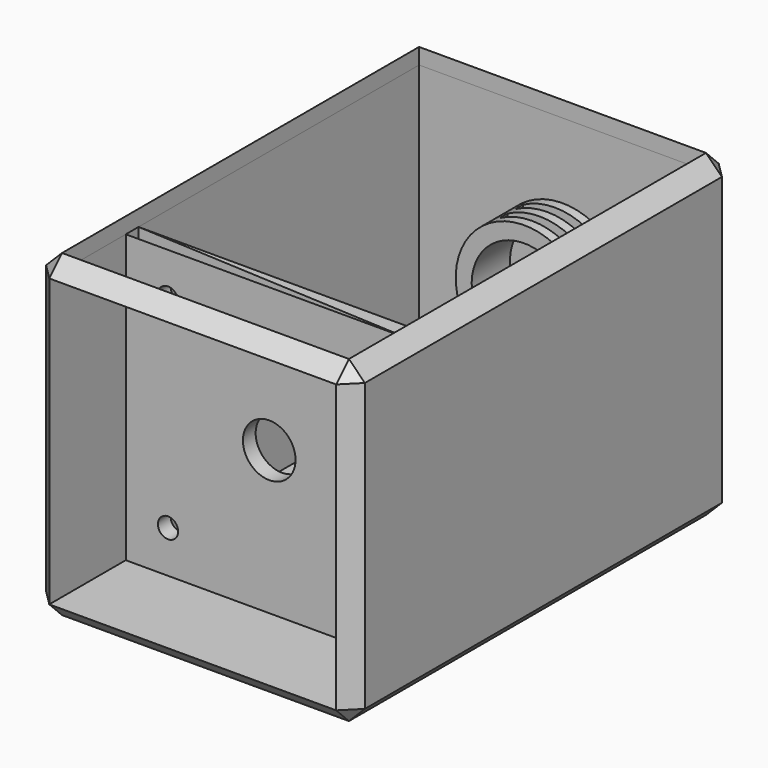
from build123d import *

# Parameters (mm, degrees)
F0_W           = 100
F0_H           = 100
F1_DEPTH       = 150
F2_W           = 90
F2_H           = 90
F3_DEPTH       = 145
F5_R           = 21.5
F5_R_2         = 16.5
F6_DEPTH       = 15
F8_DEPTH       = 21.7
F8_DEPTH_BACK  = 10
F10_W          = 3
F10_H          = 5
F11_DEPTH      = 5
F11_DEPTH_BACK = 4
F12_R          = 1
F13_DEPTH      = 15
F14_W          = 33
F14_H          = 43
F15_DEPTH      = 34
F17_DEPTH      = 130.001
F18_SIZE       = 4.99999
F19_W          = 90
F19_H          = 5
F20_DEPTH      = 90
F21_R          = 8.255
F22_DEPTH      = 5
F23_R          = 3.175
F24_DEPTH      = 5
F25_DEPTH      = 5


# Not quite as in the source:
# - a fillet or chamfer is up to 0.001 mm smaller than in the source, because OpenCascade refuses the exact size


with BuildPart() as f1:
    # F0 (on Front) → F1 (new body)
    with BuildSketch(Plane.XZ):
        Rectangle(F0_W, F0_H)
    extrude(amount=F1_DEPTH)

    # F2 (on face) → F3 (cut)
    with BuildSketch(Plane.XZ.offset(150)):
        Rectangle(F2_W, F2_H)
    extrude(amount=-F3_DEPTH, mode=Mode.SUBTRACT)

    # F5 (on face) → F6 (join)
    with BuildSketch(Plane.XZ.offset(5)):
        Circle(F5_R)
        Circle(F5_R_2, mode=Mode.SUBTRACT)
    extrude(amount=F6_DEPTH)

    # F7 (on Right) → F8 (cut, two sides)
    with BuildSketch(Plane.YZ) as f8_sk:
        Polygon((-8, 21.5), (-11, 21.5), (-11, 5), (-14, 5), (-14, 21.5), (-17, 21.5), (-17, -21.5), (-14, -21.5), (-14, 0), (-11, 0), (-11, -21.5), (-8, -21.5), align=None)
    extrude(amount=F8_DEPTH, mode=Mode.SUBTRACT)
    extrude(f8_sk.sketch, amount=-F8_DEPTH_BACK, mode=Mode.SUBTRACT)

    # F10 (on offset) → F11 (join, two sides)
    with BuildSketch(Plane.YZ.offset(21)) as f11_sk:
        with Locations((-12.5, 7.5)):
            Rectangle(F10_W, F10_H)
        with Locations((-12.5, -2.5)):
            Rectangle(F10_W, F10_H)
    extrude(amount=F11_DEPTH)
    extrude(f11_sk.sketch, amount=-F11_DEPTH_BACK)

    # F12 (on face) → F13 (cut, through all)
    with BuildSketch(Plane.XY.offset(10)):
        with Locations((23, -12.5)):
            Circle(F12_R)
    extrude(amount=-F13_DEPTH, mode=Mode.SUBTRACT)

    # F14 (on face) → F15 (join)
    with BuildSketch(Plane.XY.offset(-45)):
        with Locations((0, -41.5)):
            Rectangle(F14_W, F14_H)
    extrude(amount=F15_DEPTH)

    # F16 (on face) → F17 (cut, through all)
    with BuildSketch(Plane(origin=(0, -20, 0), x_dir=(-1, 0, 0), z_dir=(0, 1, 0))):
        with BuildLine():
            Line((12.2983738762, -11), (-12.2983738762, -11))
            ThreePointArc((-12.2983738762, -11), (0, -16.5), (12.2983738762, -11))
        make_face()
    extrude(amount=-F17_DEPTH, mode=Mode.SUBTRACT)

    # F18 (size 5 in the source; OpenCascade refuses exactly that, so slightly less here)
    f18_edges = [f1.edges().sort_by_distance(p)[0] for p in [
        (50, -75, 50),
        (-50, -75, 50),
        (0, 0, 50),
        (0, -150, 50),
        (50, -75, -50),
        (50, 0, 0),
        (50, -150, 0),
        (-50, -75, -50),
        (0, 0, -50),
        (0, -150, -50),
        (-50, 0, 0),
        (-50, -150, 0),
    ]]
    chamfer(f18_edges, length=F18_SIZE)

    # F19 (on face) → F20 (join, through all)
    with BuildSketch(Plane.XY.offset(-45)):
        with Locations((0, -117.5)):
            Rectangle(F19_W, F19_H)
    extrude(amount=F20_DEPTH)

    # F21 (on face) → F22 (cut)
    with BuildSketch(Plane.XZ.offset(120)):
        Circle(F21_R)
    extrude(amount=-F22_DEPTH, mode=Mode.SUBTRACT)

    # F23 (on face) → F24 (cut)
    with BuildSketch(Plane.XZ.offset(120)):
        with Locations((-31.75, 31.75)):
            Circle(F23_R)
        with Locations((-31.75, -31.75)):
            Circle(F23_R)
        with Locations((31.75, 31.75)):
            Circle(F23_R)
        with Locations((31.75, -31.75)):
            Circle(F23_R)
    extrude(amount=-F24_DEPTH, mode=Mode.SUBTRACT)

    # F25 (cut, through all): a face of the model
    f25_faces = [f1.faces().sort_by_distance(p)[0] for p in [
        (0, -75, 50),
    ]]
    extrude(f25_faces, amount=-F25_DEPTH, mode=Mode.SUBTRACT)


solid = f1.part
